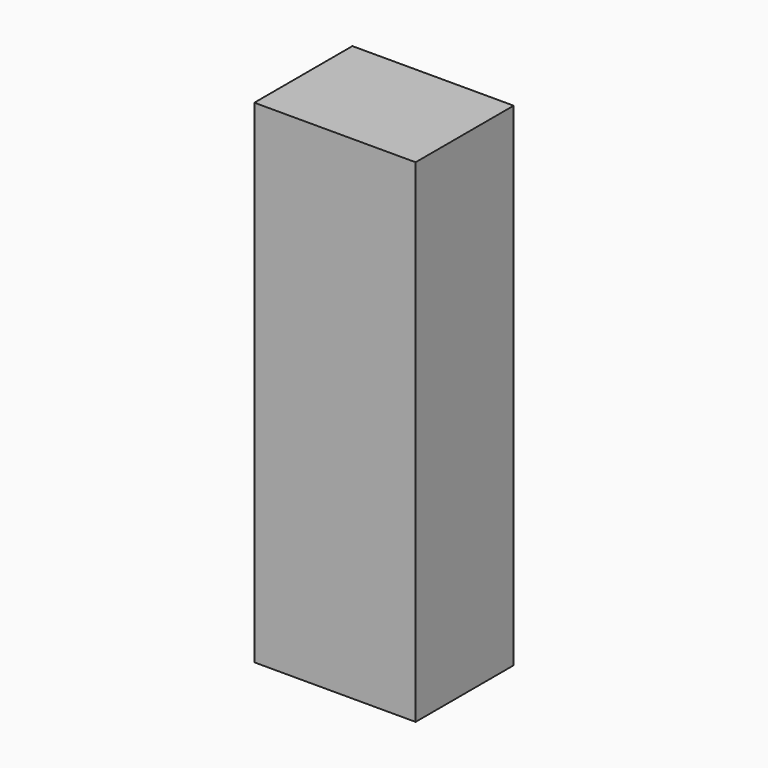
from build123d import *

# Parameters (mm, degrees)
F0_W     = 1905
F0_H     = 1447.8
F1_DEPTH = 25.4
F2_W     = 1905
F2_H     = 1447.8
F3_DEPTH = 5794.8233563


# Not quite as in the source:
# - an extrude ends at something that could not be found from the text; its depth is read off the source's solid
# - a feature of the source that left no trace in its solid (it failed there, or was rolled back) is left out


with BuildPart() as f1:
    # F0 (on Top) → F1 (new body)
    with BuildSketch(Plane.XY):
        Rectangle(F0_W, F0_H)
    extrude(amount=F1_DEPTH)

    # F2 (on face) → F3 (join, through all)
    with BuildSketch(Plane.XY.offset(25.4)):
        Rectangle(F2_W, F2_H)
    extrude(amount=F3_DEPTH)


solid = f1.part
